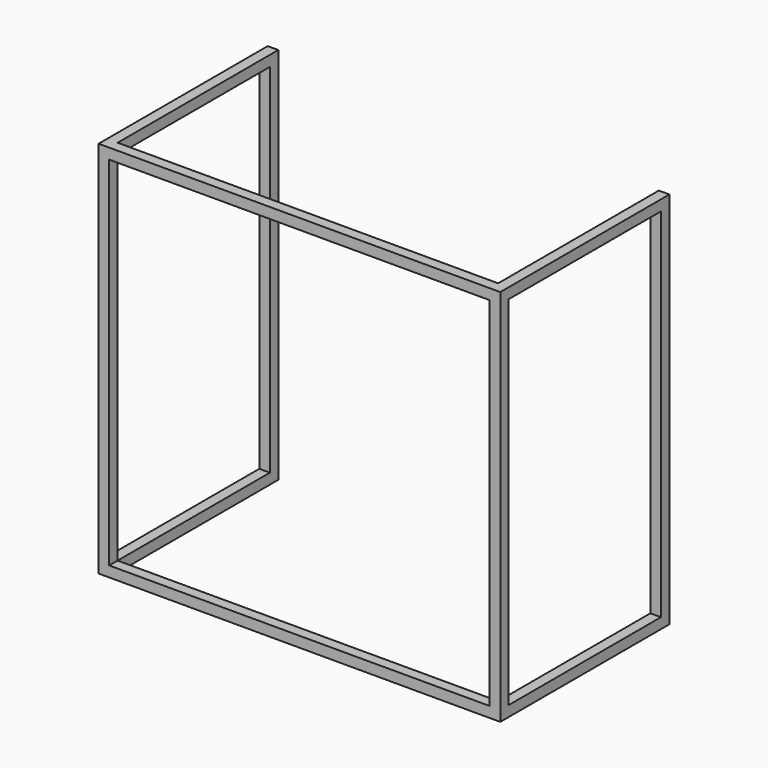
from build123d import *

# Parameters (mm, degrees)
F1_DEPTH      = 179
F2_W          = 90.0000002235
F2_H          = 169.0000002235
F3_DEPTH      = 200
F3_DEPTH_BACK = 200
F4_W          = 180.0000002235
F4_H          = 169.0000002235
F5_DEPTH      = 25


# Not quite as in the source:
# - the program builds the solid bodies; features that only make, move or delete a surface that nothing else refers to are left out


with BuildPart() as f1:
    # F0 (on Top) → F1 (new body)
    with BuildSketch(Plane.XY):
        Polygon((-74.2097248461, 100), (-74.2097248461, 0), (115.7902751539, 0), (115.7902751539, 100), (110.7902751539, 100), (110.7902751539, 5), (-69.2097248461, 5), (-69.2097248461, 100), align=None)
    extrude(amount=F1_DEPTH)

    # F2 (on face) → F3 (cut, two sides)
    with BuildSketch(Plane.YZ.offset(115.7902751539)) as f3_sk:
        with Locations((50, 89.5)):
            Rectangle(F2_W, F2_H)
    extrude(amount=F3_DEPTH, mode=Mode.SUBTRACT)
    extrude(f3_sk.sketch, amount=-F3_DEPTH_BACK, mode=Mode.SUBTRACT)

    # F4 (on face) → F5 (cut)
    with BuildSketch(Plane.XZ):
        with Locations((20.7902751539, 89.5)):
            Rectangle(F4_W, F4_H)
    extrude(amount=-F5_DEPTH, mode=Mode.SUBTRACT)


solid = f1.part
